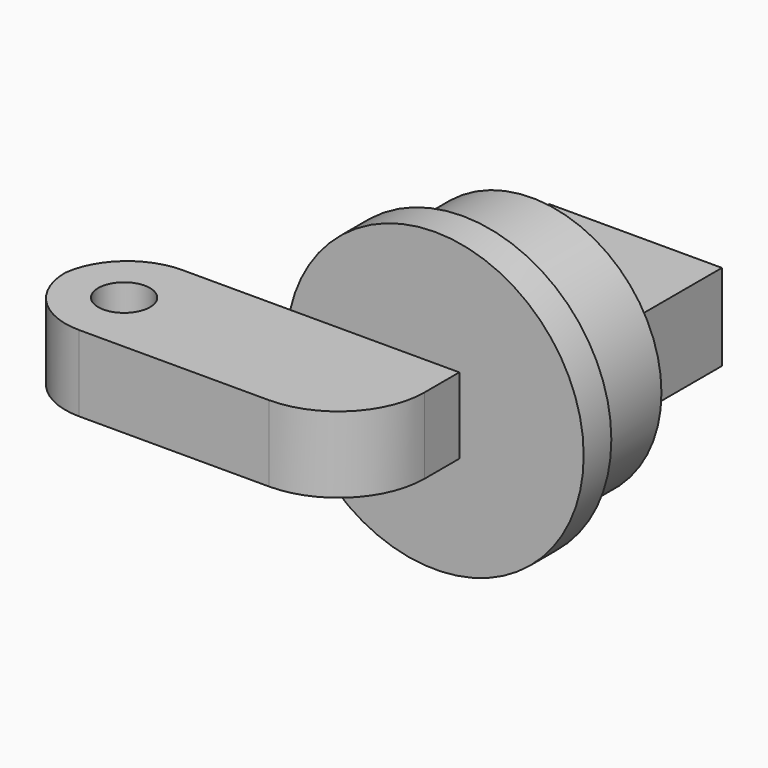
from build123d import *

# Parameters (mm, degrees)
F0_R        = 9.525
F1_DEPTH    = 6.35
F2_W        = 12.7
F2_H        = 6.35
F3_DEPTH    = 9.525
F4_R        = 10.922
F5_DEPTH    = 2.54
F6_W        = 25.4
F6_H        = 5.588
F7_DEPTH    = 9.525
F8_R        = 5.08
F9_T1_DEPTH = 30.7887812379
F10_R       = 6.35
F11_R       = 1.905
F12_DEPTH   = 13.336


# Not quite as in the source:
# - a fillet or chamfer that OpenCascade refuses, or shapes differently, is made with other operations: its cross-section is extruded or revolved along the edge and cut away or added


with BuildPart() as f1:
    # F0 (on Front) → F1 (new body)
    with BuildSketch(Plane.XZ):
        Circle(F0_R)
    extrude(amount=F1_DEPTH)

    # F2 (on face) → F3 (join)
    with BuildSketch(Plane(origin=(0, 0, 0), x_dir=(-1, 0, 0), z_dir=(0, 1, 0))):
        Rectangle(F2_W, F2_H)
    extrude(amount=F3_DEPTH)

    # F4 (on face) → F5 (join)
    with BuildSketch(Plane.XZ.offset(6.35)):
        Circle(F4_R)
    extrude(amount=F5_DEPTH)

    # F6 (on face) → F7 (join)
    with BuildSketch(Plane.XZ.offset(8.89)):
        with Locations((-10.922, -0.381)):
            Rectangle(F6_W, F6_H)
    extrude(amount=F7_DEPTH)

    # F8
    f8_edges = [f1.edges().sort_by_distance(p)[0] for p in [
        (-23.622, -18.415, -0.381),
    ]]
    fillet(f8_edges, radius=F8_R)

    # F9: fillet of radius 5.08 on 1 edges, made by hand

    # F9_s2 → F9_t1 (cut)
    with BuildSketch(Plane.XY.offset(-15.7753906189)):
        with BuildLine():
            ThreePointArc((-23.622, -13.335), (-21.9419479175, -10.16), (-18.5818437524, -8.89))
            Line((-18.5818437524, -8.89), (-23.622, -8.89))
            Line((-23.622, -8.89), (-23.622, -13.335))
        make_face()
    extrude(amount=F9_T1_DEPTH, mode=Mode.SUBTRACT)

    # F10
    f10_edges = [f1.edges().sort_by_distance(p)[0] for p in [
        (1.778, -18.415, -0.381),
    ]]
    fillet(f10_edges, radius=F10_R)

    # F11 (on face) → F12 (cut, through all)
    with BuildSketch(Plane.XY.offset(2.413)):
        with Locations((-19.05, -13.6525)):
            Circle(F11_R)
    extrude(amount=-F12_DEPTH, mode=Mode.SUBTRACT)


solid = f1.part
